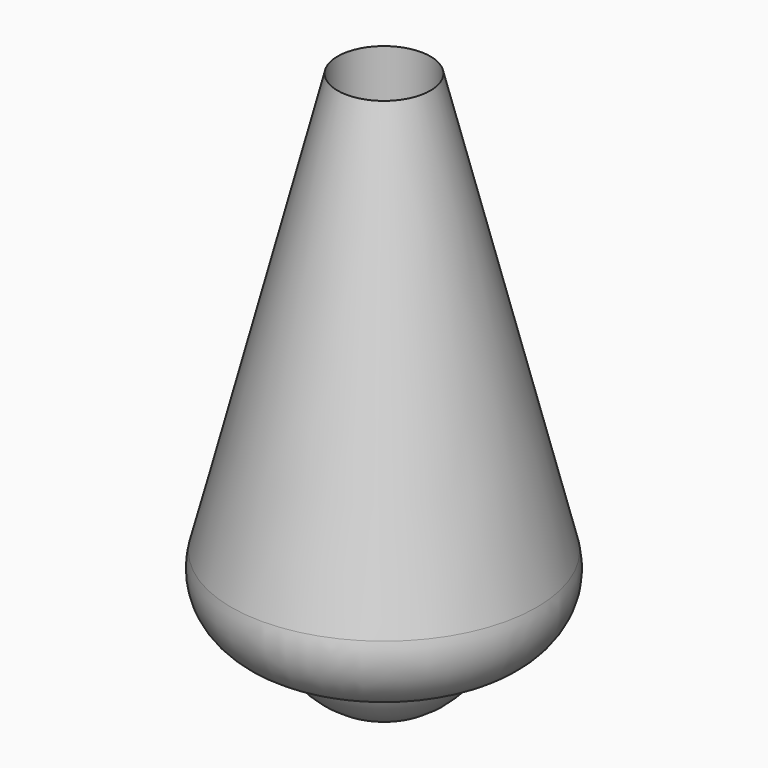
from build123d import *

# Parameters (mm, degrees)
F2_R          = 1.5
F3_DEPTH      = 3.9981844721
F3_DEPTH_BACK = 20.001


with BuildPart() as f1:
    # F0 (on Front) → F1 (revolve)
    with BuildSketch(Plane.XZ):
        with BuildLine():
            Line((-2.878140574, -1.9962841181), (-2.8287398282, -1.9962995728))
            ThreePointArc((-2.8287398282, -1.9962995728), (-1.7324339378, -3.4464032559), (0, -3.9971844721))
            Line((0, -3.9971844721), (0, 20))
            Line((0, 20), (-4.9388373396, 0.4908256009))
            ThreePointArc((-4.9388373396, 0.4908256009), (-4.6153137444, -1.1793055189), (-3.1231084445, -1.9962074819))
            Line((-3.1231084445, -1.9962074819), (-2.878140574, -1.9962841181))
        make_face()
        with BuildLine():
            ThreePointArc((-3.1231084445, -1.9962074819), (-3.0006256837, -1.9999999021), (-2.878140574, -1.9962841181))
            Line((-2.878140574, -1.9962841181), (-3.1231084445, -1.9962074819))
        make_face()
    revolve(axis=Axis((0, 0, 8.001407764), (0, 0, -1)))

    # F2 (on Top) → F3 (cut, two sides)
    with BuildSketch(Plane.XY) as f3_sk:
        Circle(F2_R)
    extrude(amount=-F3_DEPTH, mode=Mode.SUBTRACT)
    extrude(f3_sk.sketch, amount=F3_DEPTH_BACK, mode=Mode.SUBTRACT)


solid = f1.part
